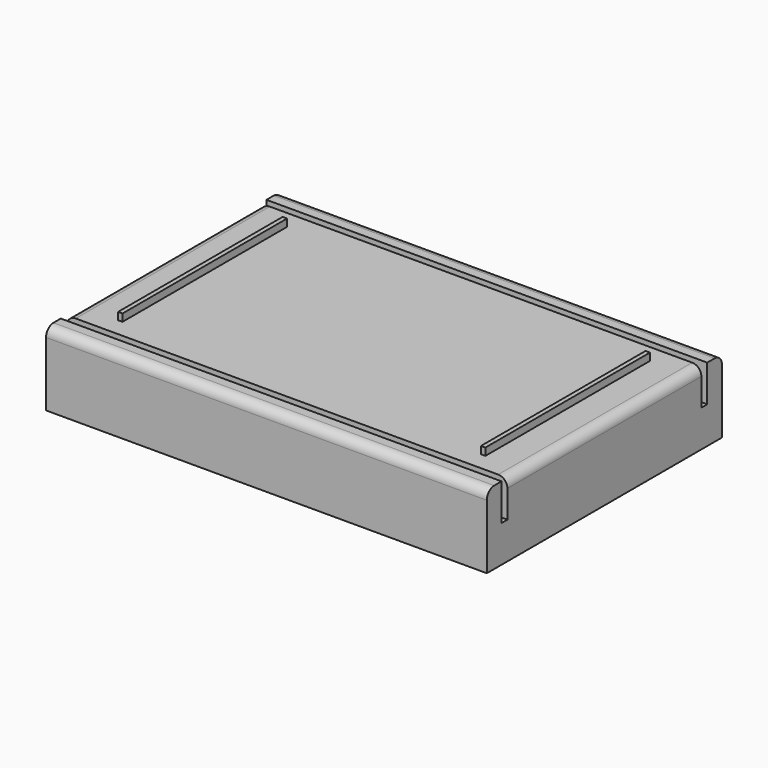
from build123d import *

# Parameters (mm, degrees)
F0_W        = 101.6
F0_H        = 25.4
F1_DEPTH    = 152.4
F2_W        = 2.54
F2_H        = 12.7
F3_DEPTH    = 152.401
F4_W        = 1.524
F4_H        = 71.12
F5_DEPTH    = 2.54
F6_R        = 3.175
F7_T        = 3.175
F7_T3_DEPTH = 158.75
F7_T5_DEPTH = 77.47
F7_T7_DEPTH = 7.874
F7_T9_DEPTH = 7.874


# Not quite as in the source:
# - a shell that OpenCascade refuses in one call is made with other operations: the cavity is built on its own and cut out


with BuildPart() as f1:
    # F0 (on Right) → F1 (new body)
    with BuildSketch(Plane.YZ):
        with Locations((50.8, 12.7)):
            Rectangle(F0_W, F0_H)
    extrude(amount=-F1_DEPTH)

    # F2 (on face) → F3 (cut, through all)
    with BuildSketch(Plane.YZ):
        with Locations((7.62, 19.05)):
            Rectangle(F2_W, F2_H)
        with Locations((93.98, 19.05)):
            Rectangle(F2_W, F2_H)
    extrude(amount=-F3_DEPTH, mode=Mode.SUBTRACT)

    # F4 (on face) → F5 (join)
    with BuildSketch(Plane.XY.offset(25.4)):
        with Locations((-138.938, 50.8)):
            Rectangle(F4_W, F4_H)
        with Locations((-13.462, 50.8)):
            Rectangle(F4_W, F4_H)
    extrude(amount=F5_DEPTH)

    # F6
    f6_edges = [f1.edges().sort_by_distance(p)[0] for p in [
        (-76.2, 0, 25.4),
        (-76.2, 101.6, 25.4),
        (0, 50.8, 25.4),
        (-152.4, 50.8, 25.4),
    ]]
    fillet(f6_edges, radius=F6_R)

    # F7: shell of thickness 3.175, made by hand


with BuildPart() as f7_core1:
    # F7_t2: copy of F1
    add(f1.part)

    # the walls: a layer under each face that stays
    f7_faces = [f7_core1.faces().sort_by_distance(p)[0] for p in [
        (-76.2, 0, 11.1125),
        (0, 50.8, 12.7),
        (-152.4, 50.8, 12.7),
        (-76.2, 4.7625, 25.4),
        (-76.2, 6.35, 19.05),
        (-76.2, 7.62, 12.7),
        (-76.2, 8.89, 19.05),
        (-76.2, 101.6, 11.1125),
        (-76.2, 92.71, 19.05),
        (-76.2, 96.8375, 25.4),
        (-76.2, 93.98, 12.7),
        (-76.2, 95.25, 19.05),
        (-76.2, 50.8, 25.4),
        (-138.176, 50.8, 26.67),
        (-138.938, 86.36, 26.67),
        (-139.7, 50.8, 26.67),
        (-138.938, 15.24, 26.67),
        (-12.7, 50.8, 26.67),
        (-13.462, 86.36, 26.67),
        (-14.224, 50.8, 26.67),
        (-13.462, 15.24, 26.67),
        (-138.938, 50.8, 27.94),
        (-13.462, 50.8, 27.94),
    ]]
    thicken(f7_faces, amount=-F7_T, mode=Mode.SUBTRACT)

    # F7_s4 → F7_t3 (cut)
    with BuildSketch(Plane.YZ.offset(-155.575)):
        Polygon((6.38175, 12.73175), (3.175, 12.7), (3.175, 9.525), (6.35, 9.525), align=None)
        Polygon((8.85825, 12.73175), (8.89, 9.525), (12.065, 9.525), (12.065, 12.7), align=None)
        Polygon((92.74175, 12.73175), (89.535, 12.7), (89.535, 9.525), (92.71, 9.525), align=None)
        Polygon((95.21825, 12.73175), (95.25, 9.525), (98.425, 9.525), (98.425, 12.7), align=None)
    extrude(amount=F7_T3_DEPTH, mode=Mode.SUBTRACT)

    # F7_s6 → F7_t5 (cut)
    with BuildSketch(Plane.XZ.offset(-89.535)):
        Polygon((-138.14425, 25.43175), (-138.176, 22.225), (-141.351, 22.225), (-141.351, 25.4), align=None)
        Polygon((-139.73175, 25.43175), (-139.7, 22.225), (-136.525, 22.225), (-136.525, 25.4), align=None)
        Polygon((-12.66825, 25.43175), (-12.7, 22.225), (-15.875, 22.225), (-15.875, 25.4), align=None)
        Polygon((-14.25575, 25.43175), (-14.224, 22.225), (-11.049, 22.225), (-11.049, 25.4), align=None)
    extrude(amount=F7_T5_DEPTH, mode=Mode.SUBTRACT)

    # F7_s8 → F7_t7 (cut)
    with BuildSketch(Plane.YZ.offset(-142.875)):
        Polygon((86.39175, 25.43175), (86.36, 22.225), (83.185, 22.225), (83.185, 25.4), align=None)
        Polygon((15.20825, 25.43175), (15.24, 22.225), (18.415, 22.225), (18.415, 25.4), align=None)
    extrude(amount=F7_T7_DEPTH, mode=Mode.SUBTRACT)

    # F7_s10 → F7_t9 (cut)
    with BuildSketch(Plane.YZ.offset(-17.399)):
        Polygon((86.39175, 25.43175), (86.36, 22.225), (83.185, 22.225), (83.185, 25.4), align=None)
        Polygon((15.20825, 25.43175), (15.24, 22.225), (18.415, 22.225), (18.415, 25.4), align=None)
    extrude(amount=F7_T9_DEPTH, mode=Mode.SUBTRACT)


with BuildPart() as f1_1:
    add(f1.part)

    # what is left inside the walls is the cavity
    f7_cavity = [f7_core1.part.solids().sort_by_distance(p)[0] for p in [
        (-100.541667, 50.8, 0.03175),
    ]]
    add(f7_cavity, mode=Mode.SUBTRACT)


solid = f1_1.part
